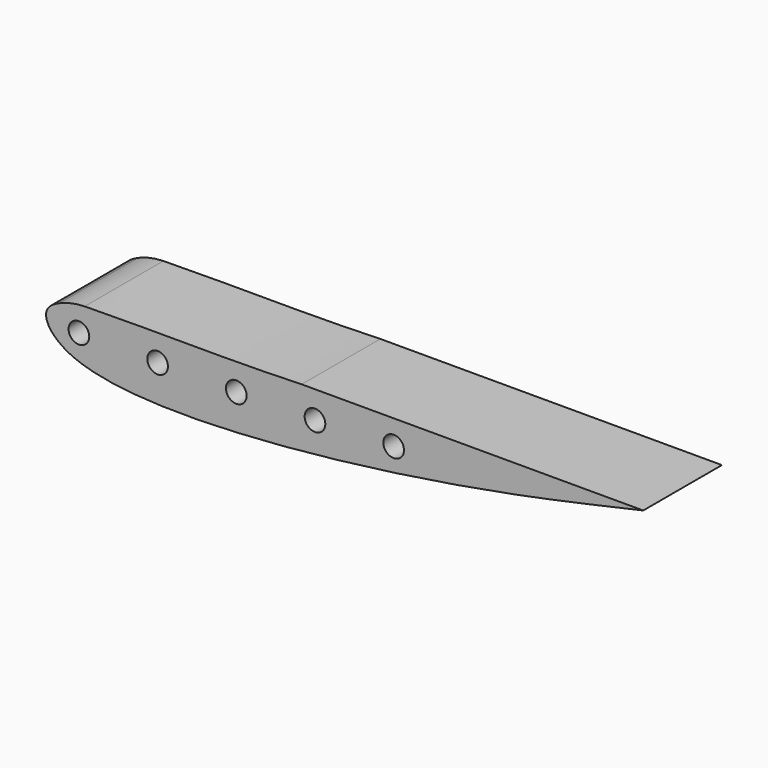
from build123d import *

# Parameters (mm, degrees)
F1_DEPTH = 10
F2_R     = 6.9
F3_R     = 1.05
F4_DEPTH = 25


with BuildPart() as f1:
    # F0 (on Front) → F1 (new body)
    with BuildSketch(Plane.XZ):
        with BuildLine():
            add(Edge.make_bspline(
                [(-21.5081513804, 15.5884723652), (-14.1544574011, 15.7776018502), (-6.8115469754, 15.5132689426), (1.56916355, 15.8104867903)],
                knots=[0, 0, 0, 0, 0.3899408074, 0.3899408074, 0.3899408074, 0.3899408074], degree=3))
            add(Edge.make_bspline(
                [(-21.5081513804, 15.5884723652), (-22.6462899262, 15.2378451635), (-25.5252357586, 14.410676063), (-20.9846389757, 7.001207284), (14.8746712309, 10.7949241928), (32.1292821065, 14.8837329452), (36.2988342287, 15.8104867903)],
                knots=[0, 0, 0, 0, 0.1188047457, 0.2585056653, 0.6845180884, 0.8898177796, 0.8898177796, 0.8898177796, 0.8898177796], degree=3))
            Line((36.2988342287, 15.8104867903), (1.56916355, 15.8104867903))
        make_face()
    extrude(amount=F1_DEPTH)

    # F2
    f2_edges = [f1.edges().sort_by_distance(p)[0] for p in [
        (-21.508151, -5, 15.588472),
    ]]
    fillet(f2_edges, radius=F2_R)

    # F3 (on face) → F4 (cut)
    with BuildSketch(Plane.XZ.offset(10)):
        with Locations((-21.0785012394, 13.0498651415)):
            Circle(F3_R)
        with Locations((2.9214987606, 13.030978851)):
            Circle(F3_R)
        with Locations((-13.0785012394, 12.9819214344)):
            Circle(F3_R)
        with Locations((-5.0785012394, 12.9561750218)):
            Circle(F3_R)
        with Locations((10.9214987606, 13.2951298729)):
            Circle(F3_R)
    extrude(amount=-F4_DEPTH, mode=Mode.SUBTRACT)


solid = f1.part
